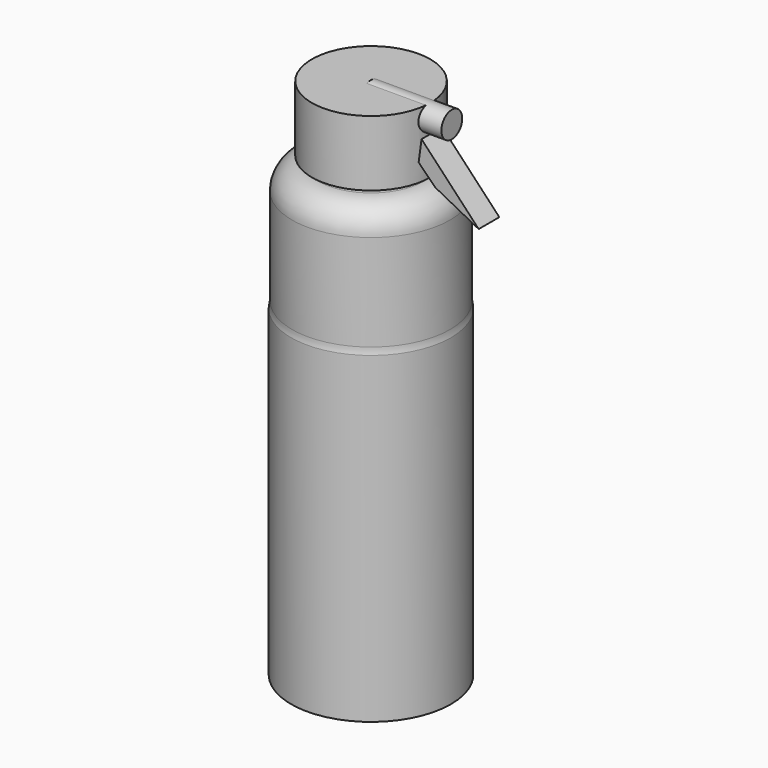
from build123d import *

# Parameters (mm, degrees)
F0_R      = 15.7315457011
F1_DEPTH  = 63.5
F2_R      = 15.5492585508
F3_DEPTH  = 25.4
F5_W      = 11.6489641368
F5_H      = 12.9090547562
F8_DEPTH  = 2.54
F9_R      = 2.5636330247
F10_DEPTH = 15.89526


# Not quite as in the source:
# - a fillet or chamfer that OpenCascade refuses, or shapes differently, is made with other operations: its cross-section is extruded or revolved along the edge and cut away or added


with BuildPart() as f1:
    # F0 (on Top) → F1 (new body)
    with BuildSketch(Plane.XY):
        Circle(F0_R)
    extrude(amount=F1_DEPTH)

    # F2 (on face) → F3 (join)
    with BuildSketch(Plane.XY.offset(63.5)):
        Circle(F2_R)
    extrude(amount=F3_DEPTH)

    # F4: fillet of radius 5.08 on 3 edges, made by hand

    # F4_s1 → F4_t2 (revolve, cut)
    with BuildSketch(Plane.XZ):
        with BuildLine():
            ThreePointArc((15.5492585508, 83.82), (14.0613609992, 87.4121024484), (10.4692585508, 88.9))
            Line((10.4692585508, 88.9), (10.4692585508, 89.0016))
            Line((10.4692585508, 89.0016), (15.6508585508, 89.0016))
            Line((15.6508585508, 89.0016), (15.6508585508, 83.82))
            Line((15.6508585508, 83.82), (15.5492585508, 83.82))
        make_face()
    revolve(axis=Axis((0, 0, 88.9), (0, 0, 1)), mode=Mode.SUBTRACT)

    # F4_s3 → F4_t4 (revolve)
    with BuildSketch(Plane.XZ):
        with BuildLine():
            ThreePointArc((15.7315457011, 63.5), (15.5950366011, 64.1681842989), (15.5492585508, 64.8486322115))
            Line((15.5492585508, 64.8486322115), (15.4476585508, 64.8486322115))
            Line((15.4476585508, 64.8486322115), (15.4476585508, 63.5))
            Line((15.4476585508, 63.5), (15.5492585508, 63.3984))
            ThreePointArc((15.5492585508, 63.3984), (15.6404021259, 63.3984), (15.6335914441, 63.4730273558))
            Line((15.6335914441, 63.4730273558), (15.7315457011, 63.5))
        make_face()
    revolve(axis=Axis((0, 0, 63.5), (0, 0, 1)))


with BuildPart() as f6:
    # F5 (on Front) → F6 (revolve)
    with BuildSketch(Plane.XZ):
        with Locations((5.8244820684, 96.3930562139)):
            Rectangle(F5_W, F5_H)
    revolve(axis=Axis((0, 0, 102.8475835919), (0, 0, 1)))

    # F7 (on Front) → F8 (join, symmetric)
    with BuildSketch(Plane.XZ):
        Polygon((23.2157874852, 85.7821851969), (11.9713721797, 97.7109819651), (11.4004518837, 93.507014215), (14.6424127743, 90.2406200767), align=None)
    extrude(amount=F8_DEPTH, both=True)

    # F9 (on Right) → F10 (join)
    with BuildSketch(Plane.YZ):
        with Locations((0, 100.4874110222)):
            Circle(F9_R)
    extrude(amount=F10_DEPTH)


solid = Compound([f1.part, f6.part])
